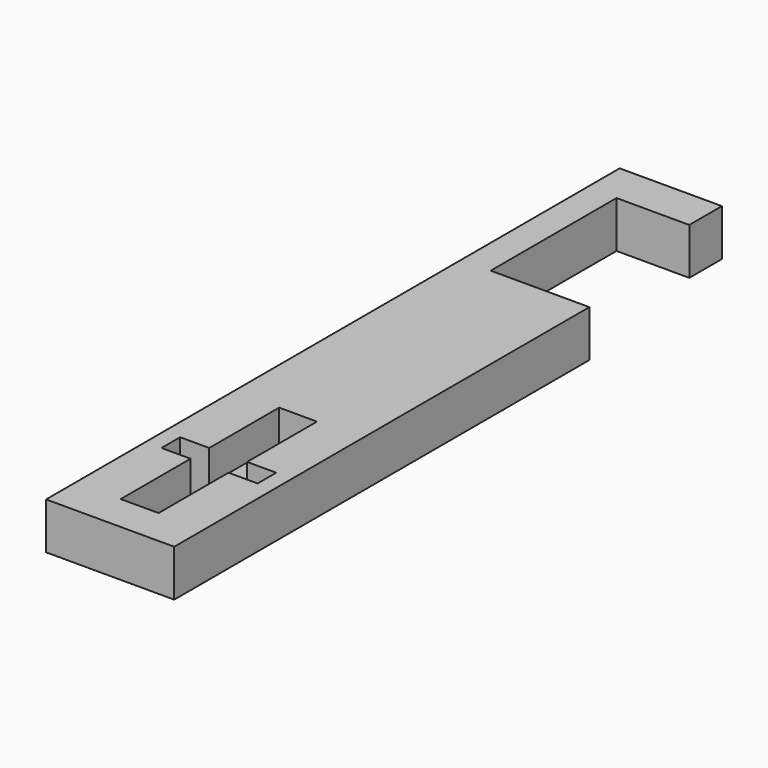
from build123d import *

# Parameters (mm, degrees)
F0_W     = 12.5
F0_H     = 7
F1_DEPTH = 8
F0_W_2   = 6.5
F0_H_2   = 15
F0_H_3   = 4
F2_DEPTH = 2.5


# Not quite as in the source:
# - a feature names something its author has since deleted; it is built from what else it names


with BuildPart() as f1:
    # F0 (on Top) → F1 (new body)
    with BuildSketch(Plane.XY):
        Polygon((-6.0006843501, 44.5469320043), (-5.9425927878, 44.5469320043), (-5.9425927878, 71.5469320043), (-5.9425927878, 78.5469320043), (-11, 78.5469320043), (-11, 44.5469320043), align=None)
        Polygon((11, -44.5469320043), (11, 44.5469320043), (1.4993156499, 44.5469320043), (-5.9425927878, 44.5469320043), (-6.0006843501, 44.5469320043), (-11, 44.5469320043), (-11, -44.5469320043), align=None)
        Polygon((-3.25, -4.2208939195), (3.25, -4.2208939195), (3.25, -19.2208939195), (8.25, -19.2208939195), (8.25, -23.2208939195), (3.25, -23.2208939195), (3.25, -38.2208939195), (-3.25, -38.2208939195), (-3.25, -23.2208939195), (-8.25, -23.2208939195), (-8.25, -19.2208939195), (-3.25, -19.2208939195), align=None, mode=Mode.SUBTRACT)
        with Locations((0.3074072122, 75.0469320043)):
            Rectangle(F0_W, F0_H)
    extrude(amount=F1_DEPTH)

    # F0 (on Top) → F2 (join)
    with BuildSketch(Plane.XY):
        with Locations((0, -11.7208939195)):
            Rectangle(F0_W_2, F0_H_2)
        with Locations((0, -21.2208939195)):
            Rectangle(F0_W_2, F0_H_3)
        with Locations((0, -30.7208939195)):
            Rectangle(F0_W_2, F0_H_2)
    extrude(amount=F2_DEPTH)


solid = f1.part
